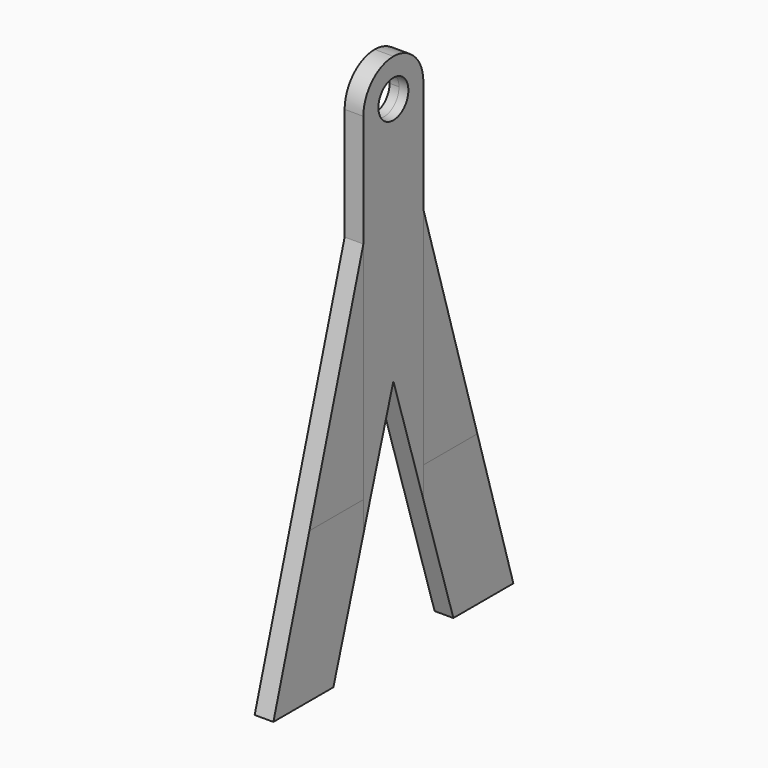
from build123d import *

# Parameters (mm, degrees)
F0_W        = 6.35
F0_H        = 25.4
F1_DEPTH    = 177.8
F0_H_2      = 38.1
F2_DEPTH    = 50.8
F4_D        = 12.7
F4_DEPTH    = 3.176
F5_D        = 12.7
F6_R        = 12.69999
F7_DEPTH    = 127
F8_T4_DEPTH = 665.7191836207
F8_T9_DEPTH = 665.7191836207
F11_DEPTH   = 25.4


# Not quite as in the source:
# - a fillet or chamfer that OpenCascade refuses, or shapes differently, is made with other operations: its cross-section is extruded or revolved along the edge and cut away or added
# - two fillets or chamfers of one size are made in one step
# - a fillet or chamfer is up to 0.001 mm smaller than in the source, because OpenCascade refuses the exact size


with BuildPart() as f1:
    # F0 (on Top) → F1 (new body)
    with BuildSketch(Plane.XY):
        Rectangle(F0_W, F0_H)
    extrude(amount=F1_DEPTH)

    # F0 (on Top) → F2 (join)
    with BuildSketch(Plane.XY):
        with Locations((0, 31.75)):
            Rectangle(F0_W, F0_H_2)
        with Locations((0, -31.75)):
            Rectangle(F0_W, F0_H_2)
    extrude(amount=F2_DEPTH)

    # F4 (through all, one way)
    with BuildSketch(Plane.YZ):
        with Locations((0, 165.1)):
            Circle(F4_D / 2)
    extrude(amount=-F4_DEPTH, mode=Mode.SUBTRACT)

    # F5 (through all)
    with Locations(Plane(origin=(0, 0, 0), x_dir=(0, 1, 0), z_dir=(-1, 0, 0))):
        with Locations((0, -165.1)):
            Hole(F5_D / 2)

    # F6 (radius 12.7 in the source; OpenCascade refuses exactly that, so slightly less here)
    f6_edges = [f1.edges().sort_by_distance(p)[0] for p in [
        (0, -12.7, 177.8),
        (0, 12.7, 177.8),
    ]]
    fillet(f6_edges, radius=F6_R)

    # F0 (on Top) → F7 (join)
    with BuildSketch(Plane.XY):
        with Locations((0, -31.75)):
            Rectangle(F0_W, F0_H_2)
        with Locations((0, 31.75)):
            Rectangle(F0_W, F0_H_2)
    extrude(amount=F7_DEPTH)

    # F8: chamfer of 38.1 x 127 on 2 edges, made by hand


with BuildPart() as f8_tool2:
    # F8_s3 → F8_t4 (new body)
    with BuildSketch(Plane.YZ.offset(332.8595918104)):
        Polygon((50.8, 0), (12.7, 127), (50.8, 127), align=None)
    extrude(amount=-F8_T4_DEPTH)

    split(bisect_by=Plane.XZ.offset(-12.7), keep=Keep.BOTTOM)


with BuildPart() as f1_1:
    add(f1.part)

    # F8_t1: cut F8_tool2
    add(f8_tool2.part, mode=Mode.SUBTRACT)


with BuildPart() as f8_tool7:
    # F8_s8 → F8_t9 (new body)
    with BuildSketch(Plane.YZ.offset(-332.8595918104)):
        Polygon((-12.7, 127), (-50.8, 0), (-50.8, 127), align=None)
    extrude(amount=F8_T9_DEPTH)

    split(bisect_by=Plane.XZ.offset(12.7), keep=Keep.TOP)


with BuildPart() as f1_2:
    add(f1_1.part)

    # F8_t6: cut F8_tool7
    add(f8_tool7.part, mode=Mode.SUBTRACT)

    # F10 (on face) → F11 (cut)
    with BuildSketch(Plane.YZ.offset(3.175)):
        Polygon((25.4, 0), (0, 80.9457584765), (-25.4, 0), align=None)
    extrude(amount=-F11_DEPTH, mode=Mode.SUBTRACT)


solid = f1_2.part
